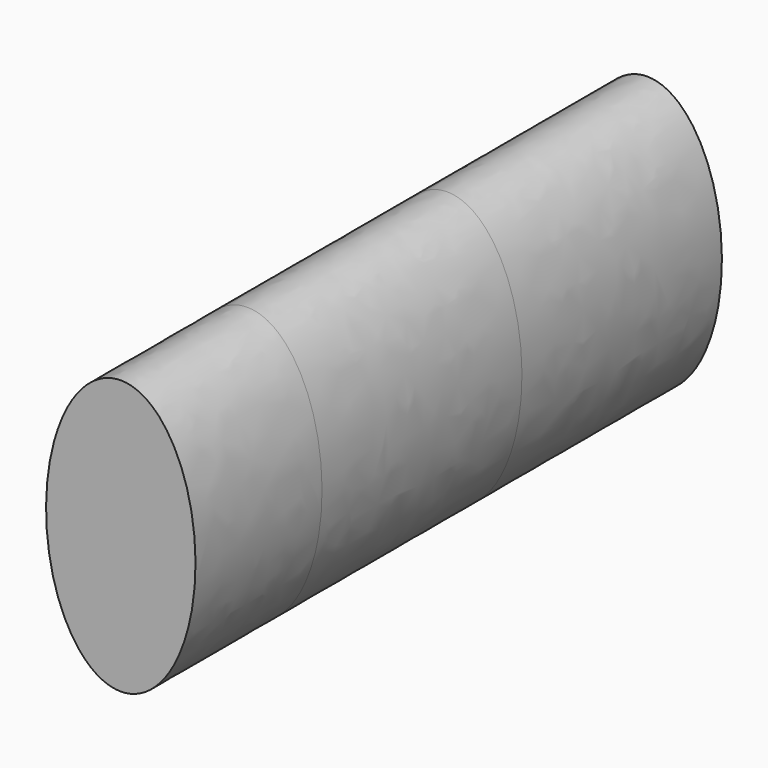
from build123d import *

# Parameters (mm, degrees)
F1_DEPTH = 40.132
F4_DEPTH = 25.4


# Not quite as in the source:
# - the program builds the solid bodies; features that only make, move or delete a surface that nothing else refers to are left out


with BuildPart() as f1:
    # F0 (on Front) → F1 (new body, symmetric)
    with BuildSketch(Plane.XZ):
        with BuildLine():
            add(Edge.make_bspline(
                [(0, -22), (20.7846096908, -22), (10.3923048454, 11), (0, 44), (-10.3923048454, 11), (-20.7846096908, -22), (0, -22)],
                knots=[0, 0, 0, 2.0943951024, 2.0943951024, 4.1887902048, 4.1887902048, 6.2831853072, 6.2831853072, 6.2831853072], degree=2, weights=[1, 0.5, 1, 0.5, 1, 0.5, 1]))
        make_face()
    extrude(amount=F1_DEPTH, both=True)

    # F4 (add): a face of the model
    f4_faces = [f1.faces().sort_by_distance(p)[0] for p in [
        (0, -40.132, 0.0533612732),
    ]]
    extrude(f4_faces, amount=F4_DEPTH)


solid = f1.part
